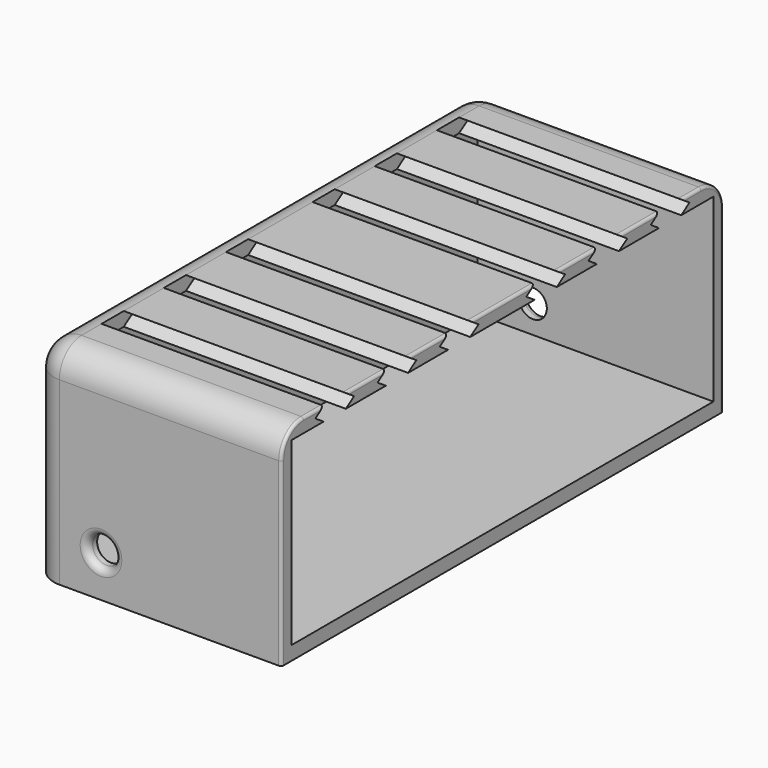
from build123d import *

# Parameters (mm, degrees)
F0_W     = 180
F0_H     = 150
F1_DEPTH = 199
F2_R     = 20
F3_R     = 20
F4_W     = 387.1927191635
F4_H     = 130
F5_DEPTH = 190
F7_DEPTH = 160
F8_R     = 10
F9_DEPTH = 264.3
F10_R    = 2
F11_R    = 5


with BuildPart() as f1:
    # F0 (on Front) → F1 (new body)
    with BuildSketch(Plane.XZ):
        with Locations((-49.0434786677, 4.1188420764)):
            Rectangle(F0_W, F0_H)
    extrude(amount=F1_DEPTH)

    # F2
    f2_edges = [f1.edges().sort_by_distance(p)[0] for p in [
        (-49.043479, -199, 79.118842),
    ]]
    fillet(f2_edges, radius=F2_R)

    # F3
    f3_edges = [f1.edges().sort_by_distance(p)[0] for p in [
        (-139.043479, -89.5, 79.118842),
    ]]
    fillet(f3_edges, radius=F3_R)

    # F4 (on Front) → F5 (cut)
    with BuildSketch(Plane.XZ):
        with Locations((64.552880914, 4.1188420764)):
            Rectangle(F4_W, F4_H)
    extrude(amount=F5_DEPTH, mode=Mode.SUBTRACT)

    # F6 (on face) → F7 (cut)
    with BuildSketch(Plane.YZ.offset(40.9565213323)):
        Polygon((-133.5333704529, 74.1188420764), (-141.0166852265, 79.1188420764), (-161.0166852265, 79.1188420764), (-168.5, 74.1188420764), (-161.0166852265, 69.1188420764), (-141.0166852265, 69.1188420764), align=None)
        Polygon((-84.9833147735, 79.1188420764), (-104.9833147735, 79.1188420764), (-112.4666295471, 74.1188420764), (-104.9833147735, 69.1188420764), (-84.9833147735, 69.1188420764), (-77.5, 74.1188420764), align=None)
        Polygon((-28.9833147735, 79.1188420764), (-48.9833147735, 79.1188420764), (-56.4666295471, 74.1188420764), (-48.9833147735, 69.1188420764), (-28.9833147735, 69.1188420764), (-21.5, 74.1188420764), align=None)
    extrude(amount=-F7_DEPTH, mode=Mode.SUBTRACT)

    # F8 (on Front) → F9 (cut)
    with BuildSketch(Plane.XZ):
        with Locations((-89.0434786677, -40.8811579236)):
            Circle(F8_R)
    extrude(amount=F9_DEPTH, mode=Mode.SUBTRACT)

    # F10
    f10_edges = [f1.edges().sort_by_distance(p)[0] for p in [
        (40.956521, -199, -5.881158),
        (40.956521, -193.142136, 73.260978),
        (40.956521, -123, 79.118842),
        (40.956521, -66.983315, 79.118842),
        (40.956521, -14.491657, 79.118842),
    ]]
    fillet(f10_edges, radius=F10_R)

    # F11
    f11_edges = [f1.edges().sort_by_distance(p)[0] for p in [
        (-99.043479, -199, -40.881158),
    ]]
    fillet(f11_edges, radius=F11_R)

    # F12: F1 across plane


with BuildPart() as f1_1:
    add(f1.part)
    add(f1.part.mirror(Plane.XZ))


solid = f1_1.part
